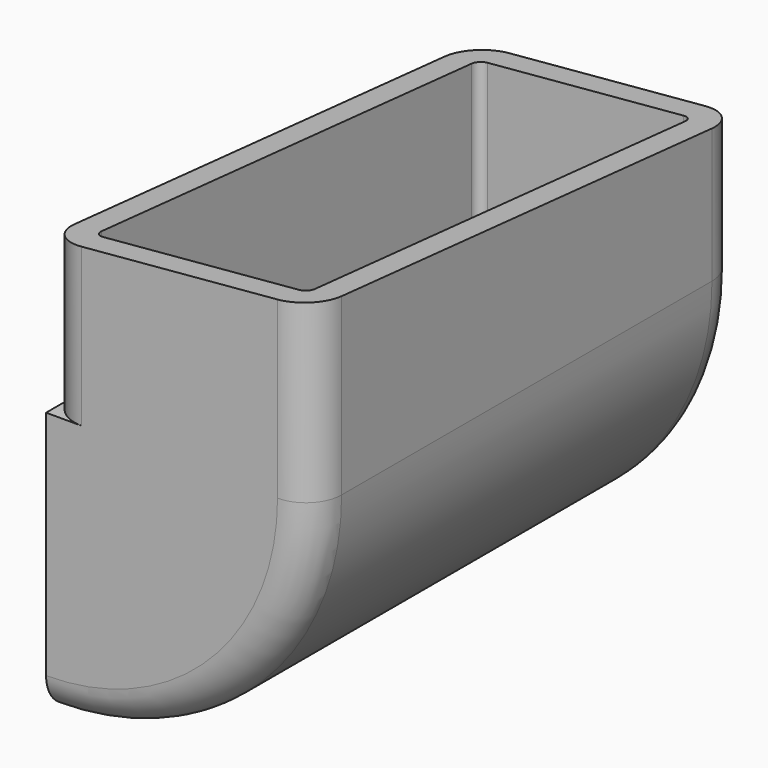
from build123d import *

# Parameters (mm, degrees)
F1_DEPTH  = 30
F2_T      = -3
F4_R      = 4
F6_DEPTH  = 20
F8_DEPTH  = 40
F9_R      = 1
F12_DEPTH = 25
F15_DEPTH = 70


# Not quite as in the source:
# - a feature of the source that left no trace in its solid (it failed there, or was rolled back) is left out


with BuildPart() as f1:
    # F0 (on Front) → F1 (new body, symmetric)
    with BuildSketch(Plane.XZ):
        with BuildLine():
            Line((0, 0), (0, -30))
            ThreePointArc((0, -30), (21.2132034356, -21.2132034356), (30, 0))
            Line((30, 0), (0, 0))
        make_face()
    extrude(amount=F1_DEPTH, both=True)

    # F2
    f2_openings = [f1.faces().sort_by_distance(p)[0] for p in [
        (15, 0, 0),
    ]]
    offset(amount=F2_T, openings=f2_openings)

    # F4
    f4_edges = [f1.edges().sort_by_distance(p)[0] for p in [
        (21.213203, -30, -21.213203),
        (21.213203, 30, -21.213203),
    ]]
    fillet(f4_edges, radius=F4_R)

    # F5 (on face) → F6 (join)
    with BuildSketch(Plane.XY):
        with BuildLine():
            Line((0, -30), (26, -30))
            ThreePointArc((26, -30), (28.8284271247, -28.8284271247), (30, -26))
            Line((30, -26), (30, 26))
            ThreePointArc((30, 26), (28.8284271247, 28.8284271247), (26, 30))
            Line((26, 30), (0, 30))
            Line((0, 30), (0, -30))
        make_face()
        Polygon((27, 26), (27, -26), (27, -27), (26, -27), (3, -27), (3, 27), (26, 27), (27, 27), align=None, mode=Mode.SUBTRACT)
    extrude(amount=F6_DEPTH)

    # F7 (on face) → F8 (cut)
    with BuildSketch(Plane(origin=(0, 0, 0), x_dir=(0, -1, 0), z_dir=(-1, 0, 0))):
        Polygon((-30, 14.7506801884), (30, 20), (-30, 20), align=None)
    extrude(amount=-F8_DEPTH, mode=Mode.SUBTRACT)

    # F9
    f9_edges = [f1.edges().sort_by_distance(p)[0] for p in [
        (3, -27, -3.547641),
        (27, -27, 9.868767),
        (27, 27, 7.506573),
        (20.124612, -27, -18),
        (3, 0, -26.832816),
        (3, 27, -5.909835),
        (20.124612, 27, -18),
    ]]
    fillet(f9_edges, radius=F9_R)

    # F11 (on offset) → F12 (cut)
    with BuildSketch(Plane.XY.offset(25)):
        with BuildLine():
            ThreePointArc((0, 26), (1.1715728753, 28.8284271247), (4, 30))
            Line((4, 30), (0, 30))
            Line((0, 30), (0, 26))
        make_face()
        with BuildLine():
            ThreePointArc((4, -30), (1.1715728753, -28.8284271247), (0, -26))
            Line((0, -26), (0, -30))
            Line((0, -30), (4, -30))
        make_face()
    extrude(amount=-F12_DEPTH, mode=Mode.SUBTRACT)

    # F14 (on face) → F15 (cut)
    with BuildSketch(Plane(origin=(0, -31.5085980719, 2.7566451349), x_dir=(1, 0, 0), z_dir=(0, -0.9961946981, 0.0871557427))):
        Polygon((26, 17.3092216794), (4, 17.3092216794), (0, 17.3092216794), (0, 14.6845617736), (30, 17.3092216794), align=None)
    extrude(amount=-F15_DEPTH, mode=Mode.SUBTRACT)


solid = f1.part
